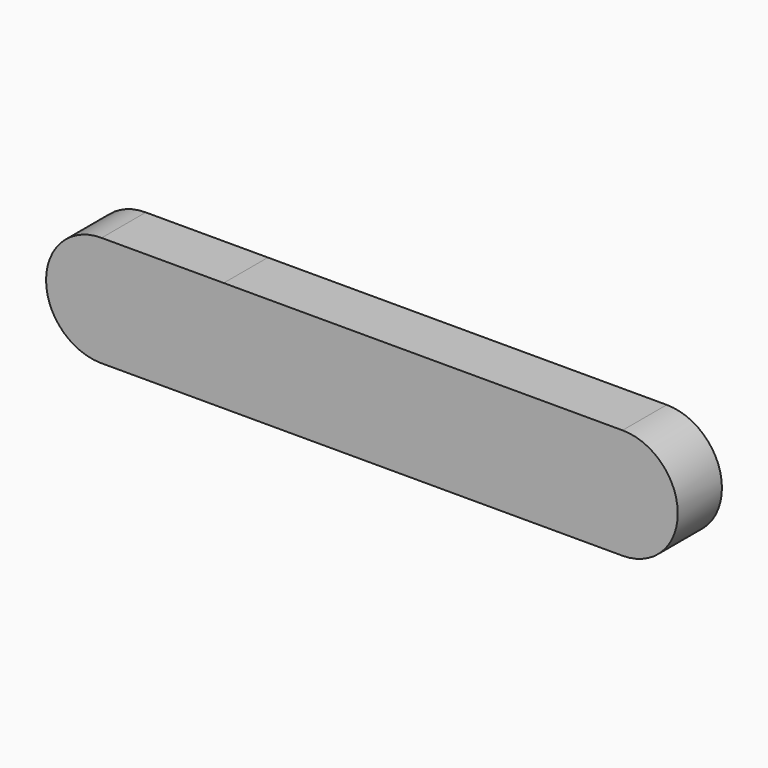
from build123d import *

# Parameters (mm, degrees)
F1_DEPTH = 12.7


# Not quite as in the source:
# - ends of sketch curves that miss each other by under 0.0002 mm in the source are joined


with BuildPart() as f1:
    # F0 (on Front) → F1 (new body)
    with BuildSketch(Plane.XZ):
        with BuildLine():
            Line((-19.0339237452, 12.7), (-38.1, 12.7))
            Line((-38.1, 12.7), (-66.1931892949, 12.6997966278))
            ThreePointArc((-66.1931892949, 12.6997966278), (-78.963911742, 0.170887308), (-66.5349535226, -12.6971318925))
            Line((-66.5349535226, -12.6971318925), (-65.9977308849, -12.6971860797))
            Line((-65.9977308849, -12.6971860797), (-38.1, -12.7))
            Line((-38.1, -12.7), (38.1, -12.7))
            Line((38.1, -12.7), (53.6455512047, -12.7))
            ThreePointArc((53.6455512047, -12.7), (66.3455512047, 0), (53.6455512047, 12.7))
            Line((53.6455512047, 12.7), (38.1, 12.7))
            Line((38.1, 12.7), (-19.0339237452, 12.7))
        make_face()
    extrude(amount=F1_DEPTH)


solid = f1.part
